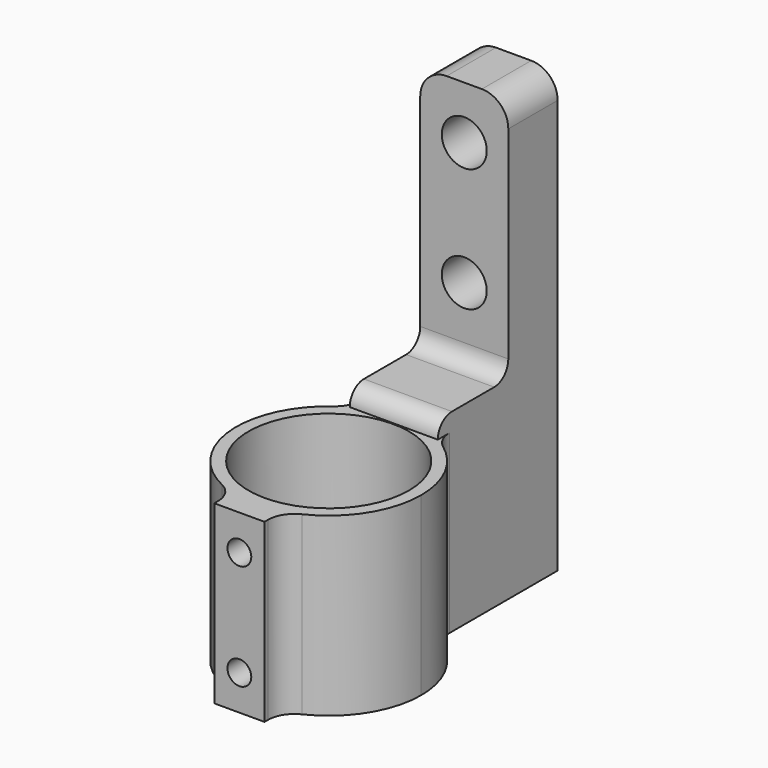
from build123d import *

# Parameters (mm, degrees)
F0_R      = 9.1
F1_DEPTH  = 20
F2_W      = 10
F2_H      = 17
F3_DEPTH  = 30
F4_W      = 10
F4_H      = 28
F5_DEPTH  = 25.4
F6_R      = 3
F7_R      = 1.99999
F8_R      = 2.5527
F9_DEPTH  = 7.001
F10_R     = 1.35255
F11_DEPTH = 3.6831519111


# Not quite as in the source:
# - a fillet or chamfer is up to 0.001 mm smaller than in the source, because OpenCascade refuses the exact size


with BuildPart() as f1:
    # F0 (on Top) → F1 (new body)
    with BuildSketch(Plane.XY):
        with BuildLine():
            ThreePointArc((2.8507034294, -10.1056167529), (8.3720483159, -6.3370976792), (10.5, 0))
            ThreePointArc((10.5, 0), (9.0208092763, 5.3735463151), (5, 9.2330926563))
            Line((5, 9.2330926563), (-5, 9.2330926563))
            ThreePointArc((-5, 9.2330926563), (-10.4357465707, -1.1598247764), (-2.8507034294, -10.1056167529))
            Line((-2.8507034294, -10.1056167529), (2.8507034294, -10.1056167529))
        make_face()
        Circle(F0_R, mode=Mode.SUBTRACT)
        with BuildLine():
            Line((-5, 9.2330926563), (5, 9.2330926563))
            ThreePointArc((5, 9.2330926563), (0, 10.5), (-5, 9.2330926563))
        make_face()
        with BuildLine():
            ThreePointArc((-5, 9.2330926563), (0, 10.5), (5, 9.2330926563))
            Line((5, 9.2330926563), (5, 26.2330926563))
            Line((5, 26.2330926563), (-5, 26.2330926563))
            Line((-5, 26.2330926563), (-5, 9.2330926563))
        make_face()
        with BuildLine():
            Line((2.8507034294, -12.6810744405), (2.8507034294, -10.1056167529))
            ThreePointArc((2.8507034294, -10.1056167529), (0, -10.5), (-2.8507034294, -10.1056167529))
            Line((-2.8507034294, -10.1056167529), (-2.8507034294, -12.6810744405))
            Line((-2.8507034294, -12.6810744405), (2.8507034294, -12.6810744405))
        make_face()
        with BuildLine():
            ThreePointArc((-2.8507034294, -10.1056167529), (0, -10.5), (2.8507034294, -10.1056167529))
            Line((2.8507034294, -10.1056167529), (-2.8507034294, -10.1056167529))
        make_face()
    extrude(amount=F1_DEPTH)

    # F2 (on face) → F3 (join)
    with BuildSketch(Plane.XY.offset(20)):
        with Locations((0, 17.7330926563)):
            Rectangle(F2_W, F2_H)
    extrude(amount=F3_DEPTH)

    # F4 (on face) → F5 (cut)
    with BuildSketch(Plane.YZ.offset(5)):
        with Locations((14.2330926563, 36)):
            Rectangle(F4_W, F4_H)
    extrude(amount=-F5_DEPTH, mode=Mode.SUBTRACT)

    # F6
    f6_edges = [f1.edges().sort_by_distance(p)[0] for p in [
        (5, 9.233093, 10),
        (-5, 9.233093, 10),
        (-5, 22.733093, 50),
        (5, 22.733093, 50),
        (2.850703, -10.105617, 10),
        (-2.850703, -10.105617, 10),
    ]]
    fillet(f6_edges, radius=F6_R)

    # F7 (radius 2 in the source; OpenCascade refuses exactly that, so slightly less here)
    f7_edges = [f1.edges().sort_by_distance(p)[0] for p in [
        (0, 9.233093, 22),
        (0, 19.233093, 22),
    ]]
    fillet(f7_edges, radius=F7_R)

    # F8 (on face) → F9 (cut, through all)
    with BuildSketch(Plane.XZ.offset(-19.2330926563)):
        with Locations((0, 44)):
            Circle(F8_R)
        with Locations((0, 30)):
            Circle(F8_R)
    extrude(amount=-F9_DEPTH, mode=Mode.SUBTRACT)

    # F10 (on face) → F11 (cut, through all)
    with BuildSketch(Plane.XZ.offset(12.6810744405)):
        with Locations((0, 16)):
            Circle(F10_R)
        with Locations((0, 4)):
            Circle(F10_R)
    extrude(amount=-F11_DEPTH, mode=Mode.SUBTRACT)


solid = f1.part
